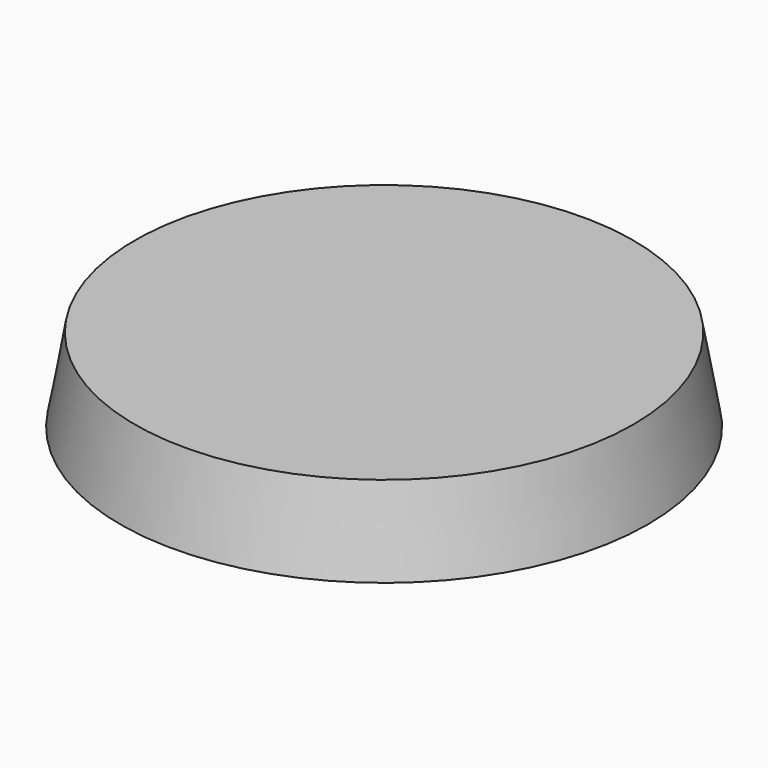
from build123d import *

# Parameters (mm, degrees)
F0_R         = 30
F1_DEPTH     = 10
F1_TAPER     = -10
F2_TEXT_SIZE = 14.1441853376
F3_DEPTH     = 1


# Not quite as in the source:
# - Text() gives the source's letters only with a copy of the font that has no kerning and outlines rounded to 1/6400 em; it was checked with that copy


with BuildPart() as f1:
    # F0 (on Top) → F1 (new body)
    with BuildSketch(Plane.XY):
        Circle(F0_R)
    extrude(amount=-F1_DEPTH, taper=F1_TAPER)

    # F2 (on face) → F3 (cut)
    with BuildSketch(Plane(origin=(0, 0, -10), x_dir=(1, 0, 0), z_dir=(0, 0, -1))):
        with Locations((-29, -5.1060585807)):
            Text('DoSpace', F2_TEXT_SIZE, font='Open Sans', text_align=(TextAlign.LEFT, TextAlign.BOTTOM))
    extrude(amount=-F3_DEPTH, mode=Mode.SUBTRACT)


solid = f1.part
